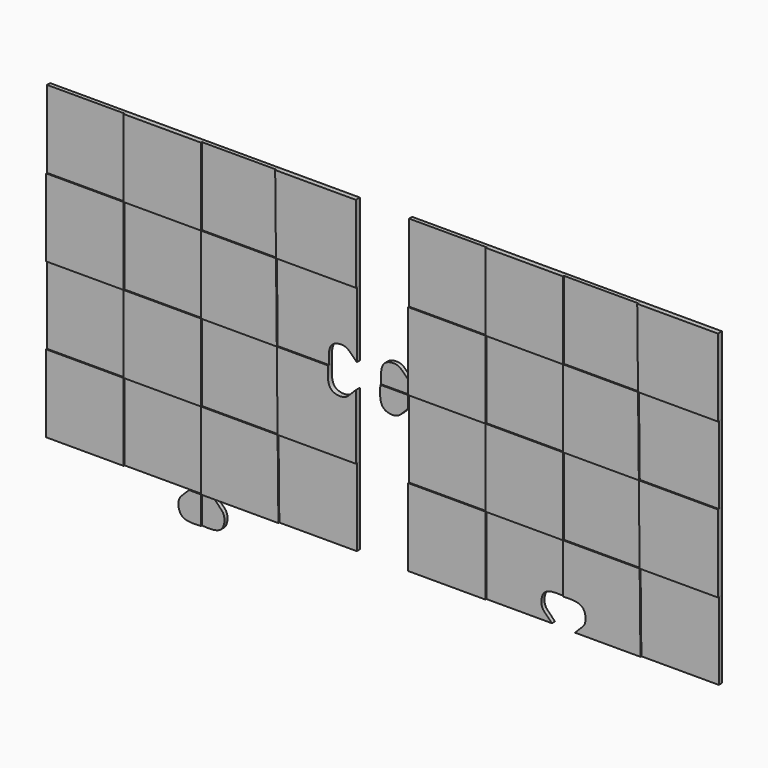
from build123d import *

# Parameters (mm, degrees)
F0_W      = 40
F0_H      = 40
F1_DEPTH  = 2
F2_DEPTH  = 2.6
F3_DEPTH  = 2
F4_DEPTH  = 2.6
F5_DEPTH  = 2.6
F6_DEPTH  = 2
F7_DEPTH  = 2
F8_DEPTH  = 2.6
F9_DEPTH  = 8.5
F10_DEPTH = 12.5


with BuildPart() as f1:
    # F0 (on Front) → F1 (new body)
    with BuildSketch(Plane.XZ):
        with Locations((-94.4291496277, 68.8439611718)):
            Rectangle(F0_W, F0_H)
    extrude(amount=F1_DEPTH)

    # F0 (on Front) → F10 (cut, symmetric)
    with BuildSketch(Plane.XZ):
        with BuildLine():
            Line((-34.4291496277, -71.1560388282), (-34.4291496277, -56.8014093116))
            add(Edge.make_bspline(
                [(-40.617107572, -71.1560388282), (-41.4295120364, -70.2954613396), (-43.2662849172, -68.3551318564), (-46.6289522951, -65.4981503471), (-45.7920089514, -58.034251825), (-40.5308587008, -56.5490574117), (-36.2922324323, -56.7152607345), (-34.897228147, -56.7428934104), (-34.4291496277, -56.8014093116)],
                knots=[0, 0, 0, 0, 0.1608830593, 0.3304410368, 0.5370562328, 0.7204150868, 0.8912918636, 1, 1, 1, 1], degree=3))
            Line((-40.617107572, -71.1560388282), (-34.4291496277, -71.1560388282))
        make_face()
        with BuildLine():
            add(Edge.make_bspline(
                [(-28.2411916833, -71.1560388282), (-27.428787219, -70.2954613396), (-25.5920143382, -68.3551318564), (-22.2293469603, -65.4981503471), (-23.066290304, -58.034251825), (-28.3274405546, -56.5490574117), (-32.5660668231, -56.7152607345), (-33.9610711084, -56.7428934104), (-34.4291496277, -56.8014093116)],
                knots=[0, 0, 0, 0, 0.1608830593, 0.3304410368, 0.5370562328, 0.7204150868, 0.8912918636, 1, 1, 1, 1], degree=3))
            Line((-34.4291496277, -56.8014093116), (-34.4291496277, -71.1560388282))
            Line((-34.4291496277, -71.1560388282), (-28.2411916833, -71.1560388282))
        make_face()
    extrude(amount=F10_DEPTH, both=True, mode=Mode.SUBTRACT)


with BuildPart() as f1b:
    # F0 (on Front) → F1, piece 2 (new body)
    with BuildSketch(Plane.XZ):
        Polygon((3.9035175741, 88.8439611718), (-34.4291496277, 88.8439611718), (-34.4291496277, 48.8439611718), (4.3203507736, 48.8439611718), align=None)
    extrude(amount=F1_DEPTH)


with BuildPart() as f1c:
    # F0 (on Front) → F1, piece 3 (new body)
    with BuildSketch(Plane.XZ):
        with Locations((-54.4291496277, 28.8439611718)):
            Rectangle(F0_W, F0_H)
    extrude(amount=F1_DEPTH)


with BuildPart() as f1d:
    # F0 (on Front) → F1, piece 4 (new body)
    with BuildSketch(Plane.XZ):
        Polygon((45.5708503723, 48.8439611718), (4.3203507736, 48.8439611718), (4.7371839732, 8.8439611718), (45.5708503723, 8.8439611718), align=None)
    extrude(amount=F1_DEPTH)


with BuildPart() as f1e:
    # F0 (on Front) → F1, piece 5 (new body)
    with BuildSketch(Plane.XZ):
        Polygon((-74.4291496277, -31.1560388282), (-74.4291496277, 8.8439611718), (-114.4291496277, 8.8439611718), (-114.4291496277, 2.6560032275), (-114.4291496277, -31.1560388282), align=None)
    extrude(amount=F1_DEPTH)


with BuildPart() as f1f:
    # F0 (on Front) → F1, piece 6 (new body)
    with BuildSketch(Plane.XZ):
        Polygon((4.7371839732, 8.8439611718), (-34.4291496277, 8.8439611718), (-34.4291496277, -31.1560388282), (5.1540171728, -31.1560388282), align=None)
    extrude(amount=F1_DEPTH)


with BuildPart() as f1g:
    # F0 (on Front) → F1, piece 7 (new body)
    with BuildSketch(Plane.XZ):
        with BuildLine():
            Line((-34.4291496277, -71.1560388282), (-34.4291496277, -56.8014093116))
            add(Edge.make_bspline(
                [(-40.617107572, -71.1560388282), (-41.4295120364, -70.2954613396), (-43.2662849172, -68.3551318564), (-46.6289522951, -65.4981503471), (-45.7920089514, -58.034251825), (-40.5308587008, -56.5490574117), (-36.2922324323, -56.7152607345), (-34.897228147, -56.7428934104), (-34.4291496277, -56.8014093116)],
                knots=[0, 0, 0, 0, 0.1608830593, 0.3304410368, 0.5370562328, 0.7204150868, 0.8912918636, 1, 1, 1, 1], degree=3))
            Line((-40.617107572, -71.1560388282), (-34.4291496277, -71.1560388282))
        make_face()
        with BuildLine():
            Line((-34.4291496277, -31.1560388282), (-74.4291496277, -31.1560388282))
            Line((-74.4291496277, -31.1560388282), (-74.4291496277, -71.1560388282))
            Line((-74.4291496277, -71.1560388282), (-40.617107572, -71.1560388282))
            add(Edge.make_bspline(
                [(-40.617107572, -71.1560388282), (-41.4295120364, -70.2954613396), (-43.2662849172, -68.3551318564), (-46.6289522951, -65.4981503471), (-45.7920089514, -58.034251825), (-40.5308587008, -56.5490574117), (-36.2922324323, -56.7152607345), (-34.897228147, -56.7428934104), (-34.4291496277, -56.8014093116)],
                knots=[0, 0, 0, 0, 0.1608830593, 0.3304410368, 0.5370562328, 0.7204150868, 0.8912918636, 1, 1, 1, 1], degree=3))
            Line((-34.4291496277, -56.8014093116), (-34.4291496277, -31.1560388282))
        make_face()
    extrude(amount=F1_DEPTH)


with BuildPart() as f1h:
    # F0 (on Front) → F1, piece 8 (new body)
    with BuildSketch(Plane.XZ):
        Polygon((45.5708503723, -31.1560388282), (5.1540171728, -31.1560388282), (5.5708503723, -71.1560388282), (45.5708503723, -71.1560388282), align=None)
    extrude(amount=F1_DEPTH)


with BuildPart() as f2:
    # F0 (on Front) → F2 (new body)
    with BuildSketch(Plane.XZ):
        with Locations((-54.4291496277, 68.8439611718)):
            Rectangle(F0_W, F0_H)
    extrude(amount=F2_DEPTH)


with BuildPart() as f2b:
    # F0 (on Front) → F2, piece 2 (new body)
    with BuildSketch(Plane.XZ):
        Polygon((45.5708503723, 88.8439611718), (3.9035175741, 88.8439611718), (4.3203507736, 48.8439611718), (45.5708503723, 48.8439611718), align=None)
    extrude(amount=F2_DEPTH)


with BuildPart() as f2c:
    # F0 (on Front) → F2, piece 3 (new body)
    with BuildSketch(Plane.XZ):
        Polygon((4.3203507736, 48.8439611718), (-34.4291496277, 48.8439611718), (-34.4291496277, 8.8439611718), (4.7371839732, 8.8439611718), align=None)
    extrude(amount=F2_DEPTH)


with BuildPart() as f2d:
    # F0 (on Front) → F2, piece 4 (new body)
    with BuildSketch(Plane.XZ):
        Polygon((-74.4291496277, 48.8439611718), (-114.4291496277, 48.8439611718), (-114.4291496277, 15.0319191161), (-114.4291496277, 8.8439611718), (-74.4291496277, 8.8439611718), align=None)
    extrude(amount=F2_DEPTH)

    # F0 (on Front) → F3 (join)
    with BuildSketch(Plane.XZ):
        with BuildLine():
            Line((-114.4291496277, 8.8439611718), (-114.4291496277, 15.0319191161))
            add(Edge.make_bspline(
                [(-114.4291496277, 15.0319191161), (-115.2897271162, 15.8443235805), (-117.2300565995, 17.6810964613), (-120.0870381088, 21.0437638392), (-127.5509366309, 20.2068204955), (-129.0361310441, 14.9456702449), (-128.8699277213, 10.7070439764), (-128.8422950455, 9.3120396911), (-128.7837791443, 8.8439611718)],
                knots=[0, 0, 0, 0, 0.1608830593, 0.3304410368, 0.5370562328, 0.7204150868, 0.8912918636, 1, 1, 1, 1], degree=3))
            Line((-128.7837791443, 8.8439611718), (-114.4291496277, 8.8439611718))
        make_face()
    extrude(amount=F3_DEPTH)


with BuildPart() as f2e:
    # F0 (on Front) → F2, piece 5 (new body)
    with BuildSketch(Plane.XZ):
        with Locations((-54.4291496277, -11.1560388282)):
            Rectangle(F0_W, F0_H)
    extrude(amount=F2_DEPTH)


with BuildPart() as f2f:
    # F0 (on Front) → F2, piece 6 (new body)
    with BuildSketch(Plane.XZ):
        Polygon((45.5708503723, 8.8439611718), (4.7371839732, 8.8439611718), (5.1540171728, -31.1560388282), (45.5708503723, -31.1560388282), align=None)
    extrude(amount=F2_DEPTH)


with BuildPart() as f2g:
    # F0 (on Front) → F2, piece 7 (new body)
    with BuildSketch(Plane.XZ):
        with Locations((-94.4291496277, -51.1560388282)):
            Rectangle(F0_W, F0_H)
    extrude(amount=F2_DEPTH)


with BuildPart() as f2h:
    # F0 (on Front) → F2, piece 8 (new body)
    with BuildSketch(Plane.XZ):
        with BuildLine():
            add(Edge.make_bspline(
                [(-28.2411916833, -71.1560388282), (-27.428787219, -70.2954613396), (-25.5920143382, -68.3551318564), (-22.2293469603, -65.4981503471), (-23.066290304, -58.034251825), (-28.3274405546, -56.5490574117), (-32.5660668231, -56.7152607345), (-33.9610711084, -56.7428934104), (-34.4291496277, -56.8014093116)],
                knots=[0, 0, 0, 0, 0.1608830593, 0.3304410368, 0.5370562328, 0.7204150868, 0.8912918636, 1, 1, 1, 1], degree=3))
            Line((-34.4291496277, -56.8014093116), (-34.4291496277, -71.1560388282))
            Line((-34.4291496277, -71.1560388282), (-28.2411916833, -71.1560388282))
        make_face()
        with BuildLine():
            Line((5.1540171728, -31.1560388282), (-34.4291496277, -31.1560388282))
            Line((-34.4291496277, -31.1560388282), (-34.4291496277, -56.8014093116))
            add(Edge.make_bspline(
                [(-28.2411916833, -71.1560388282), (-27.428787219, -70.2954613396), (-25.5920143382, -68.3551318564), (-22.2293469603, -65.4981503471), (-23.066290304, -58.034251825), (-28.3274405546, -56.5490574117), (-32.5660668231, -56.7152607345), (-33.9610711084, -56.7428934104), (-34.4291496277, -56.8014093116)],
                knots=[0, 0, 0, 0, 0.1608830593, 0.3304410368, 0.5370562328, 0.7204150868, 0.8912918636, 1, 1, 1, 1], degree=3))
            Line((-28.2411916833, -71.1560388282), (5.5708503723, -71.1560388282))
            Line((5.5708503723, -71.1560388282), (5.1540171728, -31.1560388282))
        make_face()
    extrude(amount=F2_DEPTH)


with BuildPart() as f4:
    # F0 (on Front) → F4 (new body)
    with BuildSketch(Plane.XZ):
        with BuildLine():
            Line((-114.4291496277, 2.6560032275), (-114.4291496277, 8.8439611718))
            Line((-114.4291496277, 8.8439611718), (-128.7837791443, 8.8439611718))
            add(Edge.make_bspline(
                [(-114.4291496277, 2.6560032275), (-115.2897271162, 1.8435987631), (-117.2300565995, 0.0068258823), (-120.0870381088, -3.3558414956), (-127.5509366309, -2.5188981519), (-129.0361310441, 2.7422520987), (-128.8699277213, 6.9808783672), (-128.8422950455, 8.3758826525), (-128.7837791443, 8.8439611718)],
                knots=[0, 0, 0, 0, 0.1608830593, 0.3304410368, 0.5370562328, 0.7204150868, 0.8912918636, 1, 1, 1, 1], degree=3))
        make_face()
    extrude(amount=F4_DEPTH)


with BuildPart() as f5:
    # F0 (on Front) → F5 (new body)
    with BuildSketch(Plane.XZ):
        Polygon((-141.4292120934, 88.8439611718), (-183.0965448916, 88.8439611718), (-182.679711692, 48.8439611718), (-141.4292120934, 48.8439611718), align=None)
    extrude(amount=F5_DEPTH)


with BuildPart() as f5b:
    # F0 (on Front) → F5, piece 2 (new body)
    with BuildSketch(Plane.XZ):
        with Locations((-241.4292120934, 68.8439611718)):
            Rectangle(F0_W, F0_H)
    extrude(amount=F5_DEPTH)


with BuildPart() as f5c:
    # F0 (on Front) → F5, piece 3 (new body)
    with BuildSketch(Plane.XZ):
        with Locations((-281.4292120934, 28.8439611718)):
            Rectangle(F0_W, F0_H)
    extrude(amount=F5_DEPTH)


with BuildPart() as f5d:
    # F0 (on Front) → F5, piece 4 (new body)
    with BuildSketch(Plane.XZ):
        Polygon((-182.679711692, 48.8439611718), (-221.4292120934, 48.8439611718), (-221.4292120934, 8.8439611718), (-182.2628784925, 8.8439611718), align=None)
    extrude(amount=F5_DEPTH)


with BuildPart() as f5e:
    # F0 (on Front) → F5, piece 5 (new body)
    with BuildSketch(Plane.XZ):
        with Locations((-241.4292120934, -11.1560388282)):
            Rectangle(F0_W, F0_H)
    extrude(amount=F5_DEPTH)


with BuildPart() as f5f:
    # F0 (on Front) → F5, piece 6 (new body)
    with BuildSketch(Plane.XZ):
        with BuildLine():
            Line((-155.8134579082, 8.8439611718), (-182.2628784925, 8.8439611718))
            Line((-182.2628784925, 8.8439611718), (-181.8460452929, -31.1560388282))
            Line((-181.8460452929, -31.1560388282), (-141.4292120934, -31.1560388282))
            Line((-141.4292120934, -31.1560388282), (-141.4292120934, 2.3681910971))
            add(Edge.make_bspline(
                [(-141.4292120934, 2.3681910971), (-142.2897895819, 1.5557866327), (-144.2301190652, -0.2809862481), (-147.0871005745, -3.643653626), (-154.5509990966, -2.8067102823), (-156.0361935098, 2.4544399683), (-155.869990187, 6.6930662368), (-155.8423575111, 8.0880705221), (-155.78384161, 8.5561490414)],
                knots=[0, 0, 0, 0, 0.1608830593, 0.3304410368, 0.5370562328, 0.7204150868, 0.8912918636, 1, 1, 1, 1], degree=3))
            add(Edge.make_bspline(
                [(-155.8134579082, 8.8439611718), (-155.8051568281, 8.7445772123), (-155.795437162, 8.6489038089), (-155.78384161, 8.5561490414)],
                knots=[0.9784583195, 0.9784583195, 0.9784583195, 0.9784583195, 1, 1, 1, 1], degree=3))
        make_face()
    extrude(amount=F5_DEPTH)


with BuildPart() as f5g:
    # F0 (on Front) → F5, piece 7 (new body)
    with BuildSketch(Plane.XZ):
        with Locations((-281.4292120934, -51.1560388282)):
            Rectangle(F0_W, F0_H)
    extrude(amount=F5_DEPTH)


with BuildPart() as f5h:
    # F0 (on Front) → F5, piece 8 (new body)
    with BuildSketch(Plane.XZ):
        Polygon((-181.8460452929, -31.1560388282), (-221.4292120934, -31.1560388282), (-221.4292120934, -71.1560388282), (-215.2412613873, -71.1560388282), (-181.4292120934, -71.1560388282), align=None)
    extrude(amount=F5_DEPTH)

    # F0 (on Front) → F7 (join)
    with BuildSketch(Plane.XZ):
        with BuildLine():
            Line((-215.2412613873, -71.1560388282), (-221.4292120934, -71.1560388282))
            Line((-221.4292120934, -71.1560388282), (-221.4292193317, -85.5106683448))
            add(Edge.make_bspline(
                [(-215.2412613873, -71.1560388282), (-214.428856923, -72.0166163167), (-212.5920840422, -73.9569458), (-209.2294166643, -76.8139273093), (-210.066360008, -84.2778258314), (-215.3275102585, -85.7630202447), (-219.566136527, -85.5968169218), (-220.9611408124, -85.569184246), (-221.4292193317, -85.5106683448)],
                knots=[0, 0, 0, 0, 0.1608830593, 0.3304410368, 0.5370562328, 0.7204150868, 0.8912918636, 1, 1, 1, 1], degree=3))
        make_face()
    extrude(amount=F7_DEPTH)


with BuildPart() as f6:
    # F0 (on Front) → F6 (new body)
    with BuildSketch(Plane.XZ):
        with Locations((-281.4292120934, 68.8439611718)):
            Rectangle(F0_W, F0_H)
    extrude(amount=F6_DEPTH)


with BuildPart() as f6b:
    # F0 (on Front) → F6, piece 2 (new body)
    with BuildSketch(Plane.XZ):
        Polygon((-183.0965448916, 88.8439611718), (-221.4292120934, 88.8439611718), (-221.4292120934, 48.8439611718), (-182.679711692, 48.8439611718), align=None)
    extrude(amount=F6_DEPTH)


with BuildPart() as f6c:
    # F0 (on Front) → F6, piece 3 (new body)
    with BuildSketch(Plane.XZ):
        with Locations((-241.4292120934, 28.8439611718)):
            Rectangle(F0_W, F0_H)
    extrude(amount=F6_DEPTH)


with BuildPart() as f6d:
    # F0 (on Front) → F6, piece 4 (new body)
    with BuildSketch(Plane.XZ):
        with BuildLine():
            Line((-141.4292120934, 48.8439611718), (-182.679711692, 48.8439611718))
            Line((-182.679711692, 48.8439611718), (-182.2628784925, 8.8439611718))
            Line((-182.2628784925, 8.8439611718), (-155.8134579082, 8.8439611718))
            add(Edge.make_bspline(
                [(-141.4292120934, 14.7441069857), (-142.2897895819, 15.5565114501), (-144.2301190652, 17.3932843309), (-147.0871005745, 20.7559517088), (-154.5509990966, 19.9190083651), (-156.0361935098, 14.6578581145), (-155.8777239532, 10.6164634309), (-155.8470474754, 9.2461093473), (-155.8134579082, 8.8439611718)],
                knots=[0, 0, 0, 0, 0.1608830593, 0.3304410368, 0.5370562328, 0.7204150868, 0.8912918636, 0.9784583195, 0.9784583195, 0.9784583195, 0.9784583195], degree=3))
            Line((-141.4292120934, 14.7441069857), (-141.4292120934, 48.8439611718))
        make_face()
    extrude(amount=F6_DEPTH)


with BuildPart() as f6e:
    # F0 (on Front) → F6, piece 5 (new body)
    with BuildSketch(Plane.XZ):
        Polygon((-182.2628784925, 8.8439611718), (-221.4292120934, 8.8439611718), (-221.4292120934, -31.1560388282), (-181.8460452929, -31.1560388282), align=None)
    extrude(amount=F6_DEPTH)


with BuildPart() as f6f:
    # F0 (on Front) → F6, piece 6 (new body)
    with BuildSketch(Plane.XZ):
        with Locations((-281.4292120934, -11.1560388282)):
            Rectangle(F0_W, F0_H)
    extrude(amount=F6_DEPTH)


with BuildPart() as f6g:
    # F0 (on Front) → F6, piece 7 (new body)
    with BuildSketch(Plane.XZ):
        Polygon((-221.4292120934, -31.1560388282), (-261.4292120934, -31.1560388282), (-261.4292120934, -71.1560388282), (-227.617177276, -71.1560388282), (-221.4292120934, -71.1560388282), align=None)
    extrude(amount=F6_DEPTH)


with BuildPart() as f6h:
    # F0 (on Front) → F6, piece 8 (new body)
    with BuildSketch(Plane.XZ):
        Polygon((-141.4292120934, -31.1560388282), (-181.8460452929, -31.1560388282), (-181.4292120934, -71.1560388282), (-141.4292120934, -71.1560388282), align=None)
    extrude(amount=F6_DEPTH)


with BuildPart() as f8:
    # F0 (on Front) → F8 (new body)
    with BuildSketch(Plane.XZ):
        with BuildLine():
            Line((-221.4292193317, -85.5106683448), (-221.4292120934, -71.1560388282))
            Line((-221.4292120934, -71.1560388282), (-227.617177276, -71.1560388282))
            add(Edge.make_bspline(
                [(-227.617177276, -71.1560388282), (-228.4295817404, -72.0166163167), (-230.2663546211, -73.9569458), (-233.6290219991, -76.8139273093), (-232.7920786554, -84.2778258314), (-227.5309284048, -85.7630202447), (-223.2923021363, -85.5968169218), (-221.897297851, -85.569184246), (-221.4292193317, -85.5106683448)],
                knots=[0, 0, 0, 0, 0.1608830593, 0.3304410368, 0.5370562328, 0.7204150868, 0.8912918636, 1, 1, 1, 1], degree=3))
        make_face()
    extrude(amount=F8_DEPTH)


with BuildPart() as f9_tool:
    # F0 (on Front) → F9 (new body, symmetric)
    with BuildSketch(Plane.XZ):
        with BuildLine():
            add(Edge.make_bspline(
                [(-28.2411916833, -71.1560388282), (-27.428787219, -70.2954613396), (-25.5920143382, -68.3551318564), (-22.2293469603, -65.4981503471), (-23.066290304, -58.034251825), (-28.3274405546, -56.5490574117), (-32.5660668231, -56.7152607345), (-33.9610711084, -56.7428934104), (-34.4291496277, -56.8014093116)],
                knots=[0, 0, 0, 0, 0.1608830593, 0.3304410368, 0.5370562328, 0.7204150868, 0.8912918636, 1, 1, 1, 1], degree=3))
            Line((-34.4291496277, -56.8014093116), (-34.4291496277, -71.1560388282))
            Line((-34.4291496277, -71.1560388282), (-28.2411916833, -71.1560388282))
        make_face()
        with BuildLine():
            Line((-34.4291496277, -71.1560388282), (-34.4291496277, -56.8014093116))
            add(Edge.make_bspline(
                [(-40.617107572, -71.1560388282), (-41.4295120364, -70.2954613396), (-43.2662849172, -68.3551318564), (-46.6289522951, -65.4981503471), (-45.7920089514, -58.034251825), (-40.5308587008, -56.5490574117), (-36.2922324323, -56.7152607345), (-34.897228147, -56.7428934104), (-34.4291496277, -56.8014093116)],
                knots=[0, 0, 0, 0, 0.1608830593, 0.3304410368, 0.5370562328, 0.7204150868, 0.8912918636, 1, 1, 1, 1], degree=3))
            Line((-40.617107572, -71.1560388282), (-34.4291496277, -71.1560388282))
        make_face()
    extrude(amount=F9_DEPTH, both=True)


with BuildPart() as f1g_1:
    add(f1g.part)

    # F9: cut by f9_tool
    add(f9_tool.part, mode=Mode.SUBTRACT)


with BuildPart() as f2h_1:
    add(f2h.part)

    # F9: cut by f9_tool
    add(f9_tool.part, mode=Mode.SUBTRACT)


solid = Compound([f1.part, f1b.part, f1c.part, f1d.part, f1e.part, f1f.part, f1h.part, f2.part, f2b.part, f2c.part, f2d.part, f2e.part, f2f.part, f2g.part, f4.part, f5.part, f5b.part, f5c.part, f5d.part, f5e.part, f5f.part, f5g.part, f5h.part, f6.part, f6b.part, f6c.part, f6d.part, f6e.part, f6f.part, f6g.part, f6h.part, f8.part, f1g_1.part, f2h_1.part])
